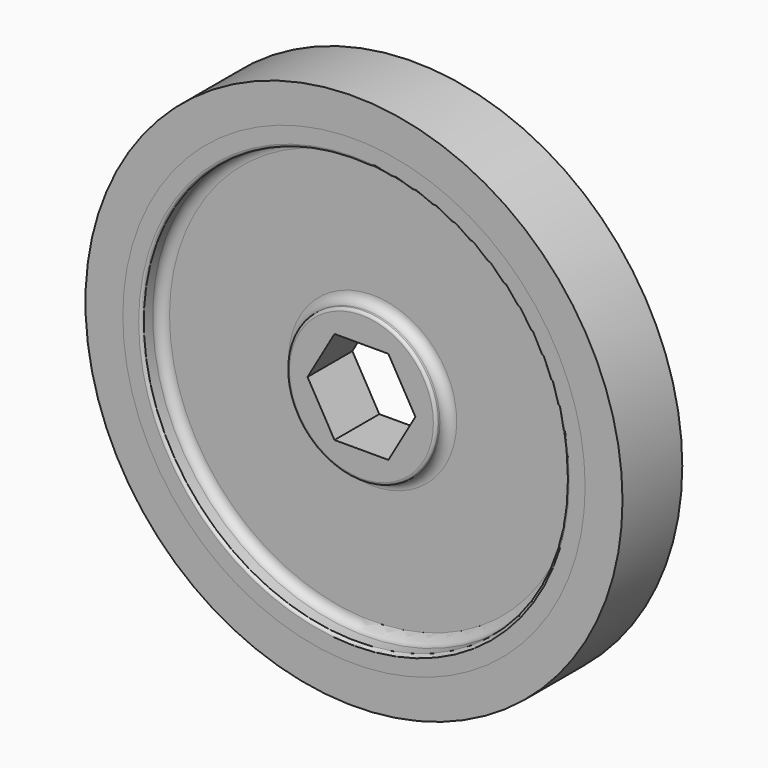
from build123d import *

# Parameters (mm, degrees)
F0_W     = 18.7325
F0_H     = 1.905
F0_W_2   = 2.54
F0_H_2   = 2.54
F3_DEPTH = 8.891
F8_R     = 1.27
F9_R     = 0.381
F10_R    = 0.381
F11_R    = 0.381


# Not quite as in the source:
# - a variable given as a bare number and used for a length is read in inches; the dataset says mm whatever the document's units were


with BuildPart() as f1:
    # F0 (on Top) → F1 (revolve)
    with BuildSketch(Plane.XY):
        Polygon((0, 3.81), (0, 0), (10.16, 0), (10.16, 1.905), (10.16, 3.81), align=None)
        with Locations((19.52625, 0.9525)):
            Rectangle(F0_W, F0_H)
        Polygon((10.16, 0), (0, 0), (0, -3.81), (10.16, -3.81), (10.16, -1.905), align=None)
        with Locations((19.52625, -0.9525)):
            Rectangle(F0_W, F0_H)
        with Locations((32.7025, -1.27)):
            Rectangle(F0_W_2, F0_H_2)
        with Locations((32.7025, 1.27)):
            Rectangle(F0_W_2, F0_H_2)
        Polygon((28.8925, 1.905), (28.8925, 0), (31.4325, 0), (31.4325, 2.54), (31.4325, 5.08), (28.8925, 5.08), align=None)
        Polygon((31.4325, 0), (28.8925, 0), (28.8925, -1.905), (28.8925, -5.08), (31.4325, -5.08), (31.4325, -2.54), align=None)
    revolve(axis=Axis((0, 1.905, 0), (0, 1, 0)))

    # F2 (on face) → F3 (cut, through all)
    with BuildSketch(Plane.XZ.offset(3.81)):
        Polygon((3.6661742094, 6.35), (-3.6661742094, 6.35), (-7.3323484187, 0), (-3.6661742094, -6.35), (3.6661742094, -6.35), (7.3323484187, 0), align=None)
    extrude(amount=-F3_DEPTH, mode=Mode.SUBTRACT)

    # F8
    f8_edges = [f1.edges().sort_by_distance(p)[0] for p in [
        (-28.8925, -1.905, 0),
        (-10.16, -1.905, 0),
    ]]
    fillet(f8_edges, radius=F8_R)

    # F9
    f9_edges = [f1.edges().sort_by_distance(p)[0] for p in [
        (-28.8925, -5.08, 0),
        (-10.16, -3.81, 0),
    ]]
    fillet(f9_edges, radius=F9_R)

    # F10
    f10_edges = [f1.edges().sort_by_distance(p)[0] for p in [
        (-31.4325, -2.54, 0),
        (-33.9725, -2.54, 0),
        (-31.4325, 2.54, 0),
        (-33.9725, 2.54, 0),
    ]]
    fillet(f10_edges, radius=F10_R)


with BuildPart() as f5:
    # F4 (on Top) → F5 (revolve)
    with BuildSketch(Plane.XY):
        Polygon((31.4325, 5.08), (31.4325, 2.54), (33.9725, 2.54), (33.9725, 0), (33.9725, -2.54), (31.4325, -2.54), (31.4325, -5.08), (36.5125, -5.08), (36.5125, 5.08), align=None)
    revolve(axis=Axis((0, 1.905, 0), (0, 1, 0)))

    # F11
    f11_edges = [f5.edges().sort_by_distance(p)[0] for p in [
        (-33.9725, 2.54, 0),
        (-31.4325, 2.54, 0),
        (-31.4325, -2.54, 0),
        (-33.9725, -2.54, 0),
    ]]
    fillet(f11_edges, radius=F11_R)


solid = Compound([f1.part, f5.part])
